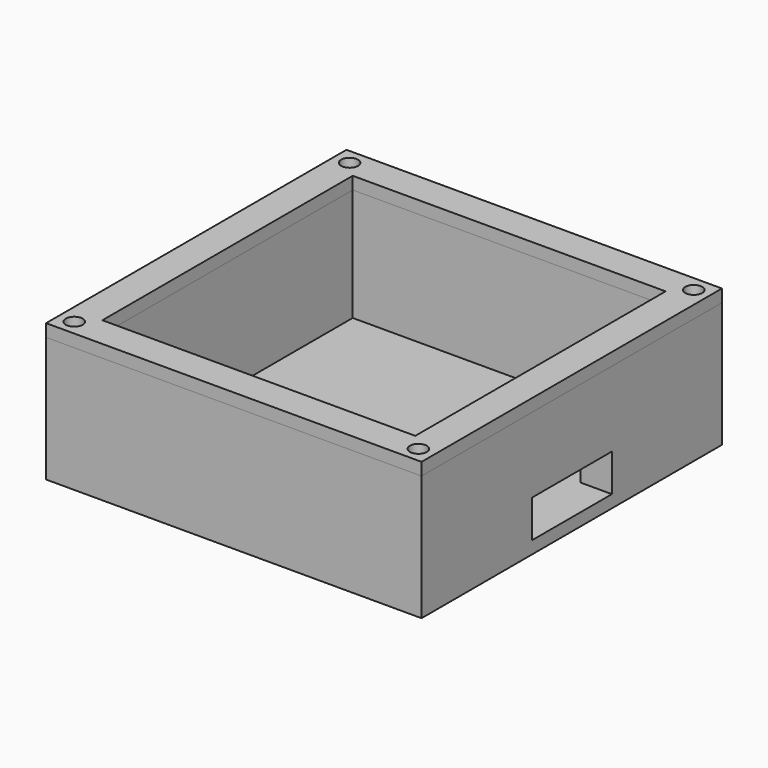
from build123d import *

# Parameters (mm, degrees)
F0_W       = 60
F0_H       = 60
F0_W_2     = 50
F0_H_2     = 50
F1_DEPTH   = 18
F2_DEPTH   = 2
F3_W       = 16
F3_H       = 6
F4_DEPTH   = 5
F5_W       = 60
F5_H       = 60
F6_DEPTH   = 2
F9_D       = 2.7
F9_DEPTH   = 4
F9_TIP     = 0.8111618357
F9_2_D     = 2.7
F9_2_DEPTH = 4
F9_2_TIP   = 0.8111618357


# Not quite as in the source:
# - a feature names something its author has since deleted; it is built from what else it names


with BuildPart() as f1:
    # F0 (on Top) → F1 (new body)
    with BuildSketch(Plane.XY):
        Rectangle(F0_W, F0_H)
        Rectangle(F0_W_2, F0_H_2, mode=Mode.SUBTRACT)
    extrude(amount=F1_DEPTH)

    # F0 (on Top) → F2 (join)
    with BuildSketch(Plane.XY):
        Rectangle(F0_W, F0_H)
        Rectangle(F0_W_2, F0_H_2, mode=Mode.SUBTRACT)
        Rectangle(F0_W_2, F0_H_2)
    extrude(amount=-F2_DEPTH)

    # F3 (on face) → F4 (cut, through all)
    with BuildSketch(Plane.YZ.offset(30)):
        with Locations((0.0201961273, 3)):
            Rectangle(F3_W, F3_H)
    extrude(amount=-F4_DEPTH, mode=Mode.SUBTRACT)

    # F9
    with Locations(Plane.XY.offset(20)):
        with Locations((-27.5, 27.5), (27.5, 27.5), (-27.5, -27.5), (27.5, -27.5)):
            Hole(F9_D / 2, depth=F9_DEPTH)
            with Locations((0, 0, -(F9_DEPTH + F9_TIP / 2))):  # 118° drill point
                Cone(0, F9_D / 2, F9_TIP, mode=Mode.SUBTRACT)


with BuildPart() as f6:
    # F5 (on face) → F6 (new body)
    with BuildSketch(Plane.XY.offset(18)):
        Rectangle(F5_W, F5_H)
        Polygon((25, 21.5), (25, 17.5), (25, -17.5), (25, -21.5), (25, -25), (-25, -25), (-25, -21.5), (-25, -17.5), (-25, 17.5), (-25, 21.5), (-25, 25), (25, 25), align=None, mode=Mode.SUBTRACT)
    extrude(amount=F6_DEPTH)

    # F9#2
    with Locations(Plane.XY.offset(20)):
        with Locations((-27.5, 27.5), (27.5, 27.5), (-27.5, -27.5), (27.5, -27.5)):
            Hole(F9_2_D / 2, depth=F9_2_DEPTH)
            with Locations((0, 0, -(F9_2_DEPTH + F9_2_TIP / 2))):  # 118° drill point
                Cone(0, F9_2_D / 2, F9_2_TIP, mode=Mode.SUBTRACT)


solid = Compound([f1.part, f6.part])
